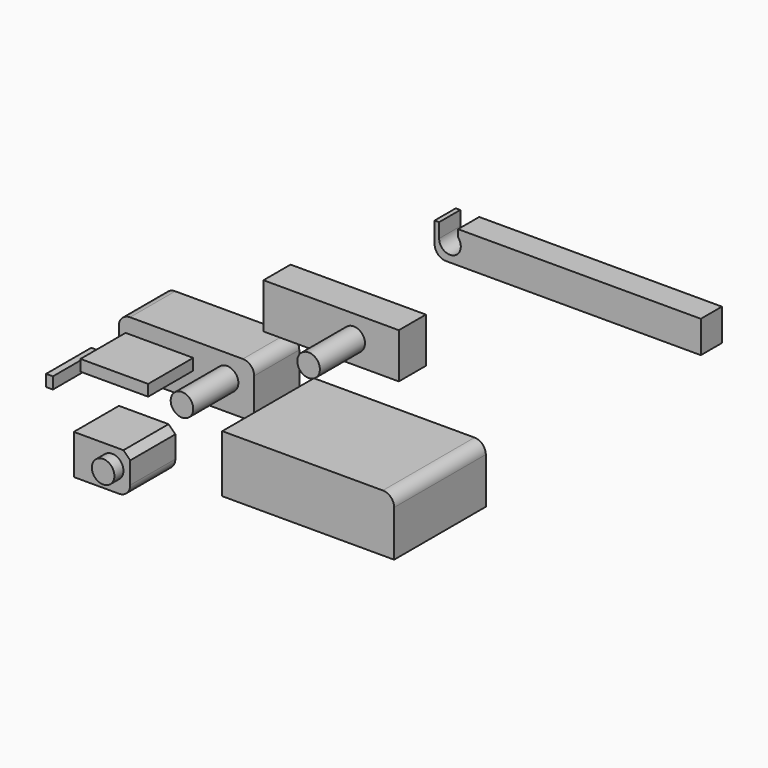
from build123d import *

# Parameters (mm, degrees)
F0_W      = 38.1
F0_H      = 25.4
F1_DEPTH  = 25.4
F3_DEPTH  = 25.4
F5_W      = 60
F5_H      = 20
F6_DEPTH  = 15
F7_R      = 5
F8_DEPTH  = 25
F9_W      = 60
F9_H      = 23.0075153246
F10_DEPTH = 25
F9_W_2    = 3.0239969492
F9_H_2    = 5.1660002209
F9_W_3    = 25
F9_H_3    = 17.6400020719
F11_R     = 5
F13_W     = 30
F13_H     = 5
F14_DEPTH = 25
F15_R     = 5
F16_DEPTH = 5
F17_SIZE  = 3
F18_R     = 5
F19_R     = 5
F20_DEPTH = 25
F21_R     = 5
F22_W     = 118
F22_H     = 14.2
F23_DEPTH = 11.7
F25_DEPTH = 25
F26_R     = 5


# Not quite as in the source:
# - the program builds the solid bodies; features that only make, move or delete a surface that nothing else refers to are left out


with BuildPart() as f1:
    # F0 (on Front) → F1 (new body)
    with BuildSketch(Plane.XZ):
        with Locations((-19.05, 12.7)):
            Rectangle(F0_W, F0_H)
        with Locations((19.05, 12.7)):
            Rectangle(F0_W, F0_H)
    extrude(amount=F1_DEPTH)

    # F3 (add): a face of the model
    f3_faces = [f1.faces().sort_by_distance(p)[0] for p in [
        (0, -25.4, 12.7),
    ]]
    extrude(f3_faces, amount=F3_DEPTH)

    # F21
    f21_edges = [f1.edges().sort_by_distance(p)[0] for p in [
        (38.1, -25.4, 25.4),
    ]]
    fillet(f21_edges, radius=F21_R)


with BuildPart() as f6:
    # F5 (on Front) → F6 (new body)
    with BuildSketch(Plane.XZ):
        with Locations((-18.4568141215, 56.381771341)):
            Rectangle(F5_W, F5_H)
    extrude(amount=F6_DEPTH)

    # F7 (on face) → F8 (join)
    with BuildSketch(Plane.XZ.offset(15)):
        with Locations((-8.4568141215, 56.381771341)):
            Circle(F7_R)
    extrude(amount=F8_DEPTH)


with BuildPart() as f10:
    # F9 (on Front) → F10 (new body)
    with BuildSketch(Plane.XZ):
        with Locations((-74.5920035988, 27.8460001573)):
            Rectangle(F9_W, F9_H)
    extrude(amount=F10_DEPTH)

    # F11
    f11_edges = [f10.edges().sort_by_distance(p)[0] for p in [
        (-104.592004, -12.5, 39.349758),
        (-104.592004, -12.5, 16.342242),
        (-44.592004, -12.5, 39.349758),
    ]]
    fillet(f11_edges, radius=F11_R)

    # F13 (on face) → F14 (join)
    with BuildSketch(Plane.XZ.offset(25)):
        with Locations((-86.5920035988, 30.1169776731)):
            Rectangle(F13_W, F13_H)
    extrude(amount=F14_DEPTH)


with BuildPart() as f10b:
    # F9 (on Front) → F10, piece 2 (new body)
    with BuildSketch(Plane.XZ):
        with Locations((-135.3240087628, 2.5830001105)):
            Rectangle(F9_W_2, F9_H_2)
    extrude(amount=F10_DEPTH)


with BuildPart() as f10c:
    # F9 (on Front) → F10, piece 3 (new body)
    with BuildSketch(Plane.XZ):
        with Locations((-112.0400026441, -22.3020017147)):
            Rectangle(F9_W_3, F9_H_3)
    extrude(amount=F10_DEPTH)

    # F15 (on face) → F16 (join)
    with BuildSketch(Plane.XZ.offset(25)):
        with Locations((-107.5400026441, -21.4820006788)):
            Circle(F15_R)
    extrude(amount=F16_DEPTH)

    # F17
    f17_edges = [f10c.edges().sort_by_distance(p)[0] for p in [
        (-99.540003, -12.5, -13.482001),
    ]]
    chamfer(f17_edges, length=F17_SIZE)

    # F18
    f18_edges = [f10c.edges().sort_by_distance(p)[0] for p in [
        (-99.540003, -12.5, -31.122003),
    ]]
    fillet(f18_edges, radius=F18_R)


with BuildPart() as f20:
    # F19 (on face) → F20 (new body)
    with BuildSketch(Plane.XZ.offset(25)):
        with Locations((-56.5920035988, 29.3497578196)):
            Circle(F19_R)
    extrude(amount=F20_DEPTH)


with BuildPart() as f23:
    # F22 (on Front) → F23 (new body)
    with BuildSketch(Plane.XZ):
        with Locations((83.7810058147, 105.068490946)):
            Rectangle(F22_W, F22_H)
    extrude(amount=F23_DEPTH)

    # F24 (on face) → F25 (cut)
    with BuildSketch(Plane.XZ.offset(11.7)):
        with BuildLine():
            ThreePointArc((26.7810058147, 105.768490946), (31.5810058147, 100.968490946), (36.3810058147, 105.768490946))
            ThreePointArc((36.3810058147, 105.768490946), (36.0709946788, 107.4655472209), (35.1810058147, 108.9433925193))
            ThreePointArc((35.1810058147, 108.9433925193), (29.8839495398, 110.2584798102), (26.7810058147, 105.768490946))
        make_face()
        with BuildLine():
            ThreePointArc((26.7810058147, 105.768490946), (29.8839495398, 110.2584798102), (35.1810058147, 108.9433925193))
            Line((35.1810058147, 108.9433925193), (35.1810058147, 112.168490946))
            Line((35.1810058147, 112.168490946), (26.7810058147, 112.168490946))
            Line((26.7810058147, 112.168490946), (26.7810058147, 105.768490946))
        make_face()
    extrude(amount=-F25_DEPTH, mode=Mode.SUBTRACT)

    # F26
    f26_edges = [f23.edges().sort_by_distance(p)[0] for p in [
        (24.781006, -5.85, 97.968491),
    ]]
    fillet(f26_edges, radius=F26_R)


solid = Compound([f1.part, f6.part, f10.part, f10b.part, f10c.part, f20.part, f23.part])
